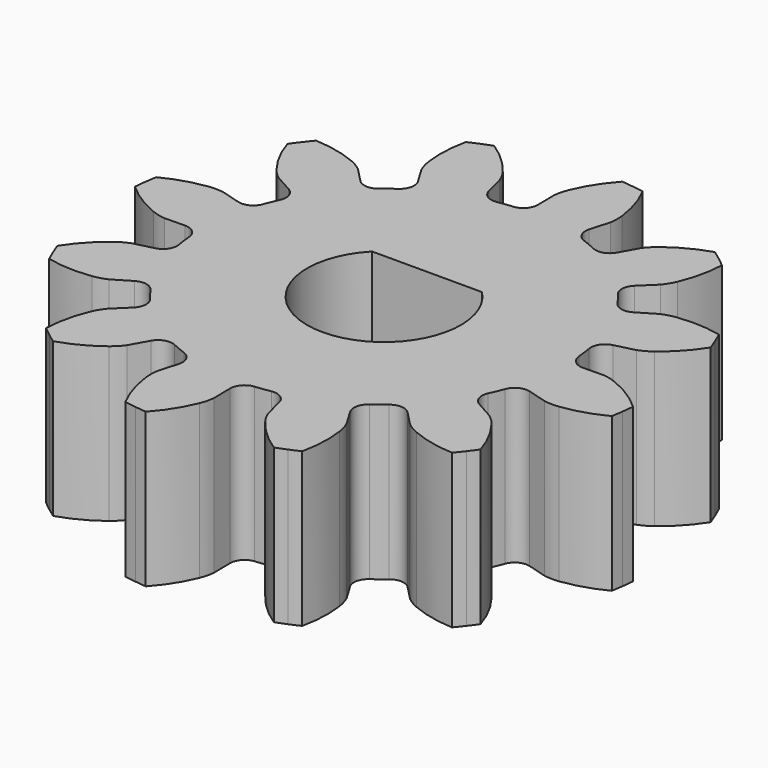
from build123d import *

# Parameters (mm, degrees)
F1_R            = 5.9375
F2_DEPTH        = 5
F4_DEPTH        = 5.001
F6_DEPTH        = 5
F6_COPIES_COUNT = 12


# Not quite as in the source:
# - a pattern or mirror of a feature is missing from the dataset's text; its kind, count and spacing are read off the source's solid


with BuildPart() as f2:
    # F1 (on Top) → F2 (new body)
    with BuildSketch(Plane.XY):
        Circle(F1_R)
    extrude(amount=F2_DEPTH)

    # F3 (on face) → F4 (cut, through all)
    with BuildSketch(Plane.XY.offset(5)):
        with BuildLine():
            Line((1.7853571071, 1.75), (-1.7853571071, 1.75))
            ThreePointArc((-1.7853571071, 1.75), (0, -2.5), (1.7853571071, 1.75))
        make_face()
    extrude(amount=-F4_DEPTH, mode=Mode.SUBTRACT)

    # F5 (on Top) → F6 (join)
    with BuildSketch(Plane.XY):
        with BuildLine():
            ThreePointArc((1.1453723021, 8.6747116546), (0.9598655071, 8.6971925475), (0.7739209425, 8.7157068775))
            ThreePointArc((0.7739209425, 8.7157068775), (0.3320811824, 8.1427896818), (0, 7.5))
            ThreePointArc((0, 7.5), (0.9817476875, 7.4354671325), (1.9466007101, 7.2429790608))
            ThreePointArc((1.9466007101, 7.2429790608), (1.7927337501, 7.9499312837), (1.514734402, 8.617892996))
            ThreePointArc((1.514734402, 8.617892996), (1.3303567226, 8.6482744516), (1.1453723021, 8.6747116546))
        make_face()
        with BuildLine():
            ThreePointArc((1.9466007101, 7.2429790608), (0.9817476875, 7.4354671325), (0, 7.5))
            ThreePointArc((0, 7.5), (-0.0726747398, 7.2774580305), (-0.112681698, 7.0467937956))
            Line((-0.112681698, 7.0467937956), (-0.1021514335, 6.3882609202))
            ThreePointArc((-0.1021514335, 6.3882609202), (-0.2224148098, 6.0671975347), (-0.5290726248, 5.9138809937))
            ThreePointArc((-0.5290726248, 5.9138809937), (0.7772169193, 5.8864114799), (2.0458702513, 5.5738964078))
            ThreePointArc((2.0458702513, 5.5738964078), (1.7895142453, 5.8015509166), (1.7567031916, 6.1428256036))
            Line((1.7567031916, 6.1428256036), (1.9377926647, 6.7760578179))
            ThreePointArc((1.9377926647, 6.7760578179), (1.9590248784, 7.0092009908), (1.9466007101, 7.2429790608))
        make_face()
    f6 = extrude(amount=F6_DEPTH)

    # F6_copies: F6 ×12 about axis
    f6_copies_axis = Axis((0, 0, 0), (0, 0, 1))
    for i in range(1, F6_COPIES_COUNT):
        add(f6.rotate(f6_copies_axis, i * 360 / F6_COPIES_COUNT))


solid = f2.part
